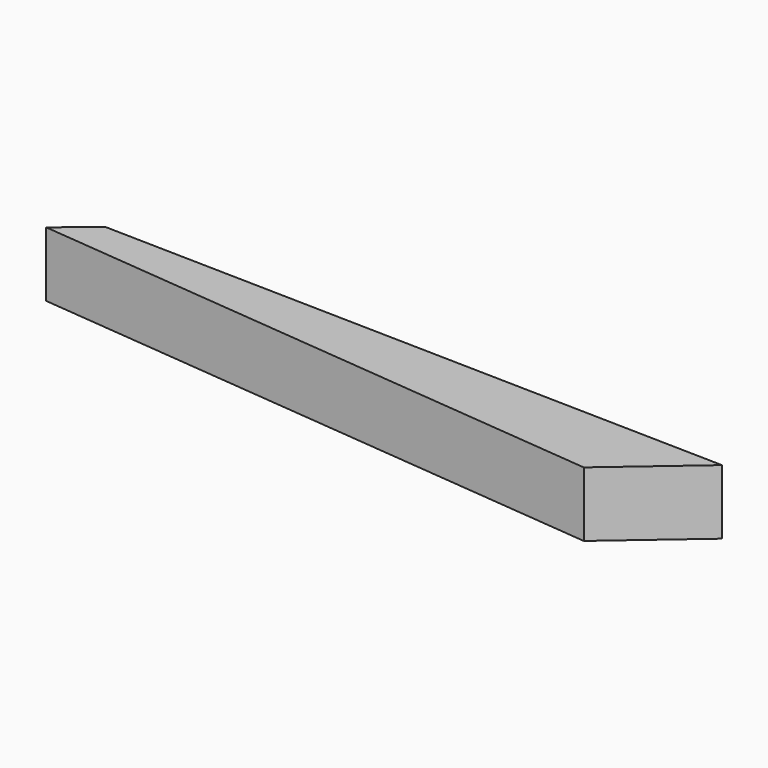
from build123d import *

# Parameters (mm, degrees)
F1_DEPTH = 25.4


# Not quite as in the source:
# - ends of sketch curves that miss each other by under 0.0002 mm in the source are joined


with BuildPart() as f1:
    # F0 (on Top) → F1 (new body)
    with BuildSketch(Plane.XY):
        Polygon((-136.5497410297, -65.4802620411), (91.5099680424, -86.9463980198), (123.5991120338, -59.3310184777), (-122.4297434092, -53.9425499737), align=None)
    extrude(amount=F1_DEPTH)


solid = f1.part
